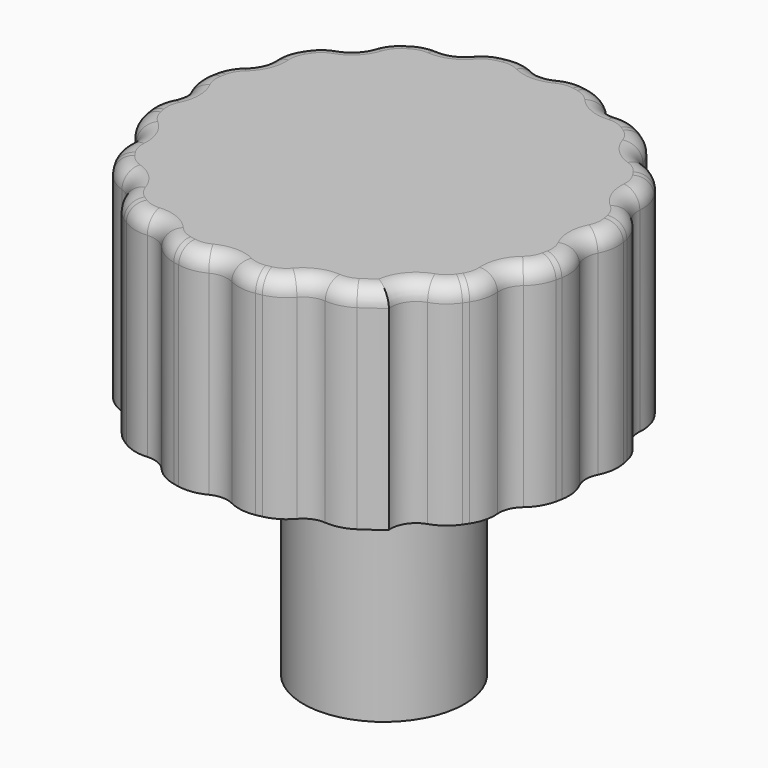
from build123d import *

# Parameters (mm, degrees)
F3_R           = 25
F4_DEPTH       = 25
F5_R           = 9.5
F6_DEPTH       = 28
F8_DEPTH       = 15
F9_R           = 3
F10_DEPTH      = 25
F11_COUNT      = 16
F13_R          = 5
F14_T4_ANGLE   = 1.6121793849
F14_T6_ANGLE   = 53.896069647
F14_T8_ANGLE   = 37.3919452447
F14_T10_ANGLE  = 37.3919452447
F14_T12_ANGLE  = 1.6121793849
F14_T14_ANGLE  = 37.3919452447
F14_T16_ANGLE  = 37.3919452447
F14_T18_ANGLE  = 53.896069647
F14_T20_ANGLE  = 53.896069647
F14_T22_ANGLE  = 37.3919452447
F14_T24_ANGLE  = 37.3919452447
F14_T26_ANGLE  = 1.6121793849
F14_T28_ANGLE  = 1.6121793849
F14_T30_ANGLE  = 37.3919452447
F14_T32_ANGLE  = 37.3919452447
F14_T34_ANGLE  = 53.896069647
F14_T36_ANGLE  = 172.9885237531
F14_T38_ANGLE  = 37.3919452447
F14_T40_ANGLE  = 18.2008968181
F14_T42_ANGLE  = 1.6121793849
F14_T44_ANGLE  = 37.3919452447
F14_T46_ANGLE  = 37.3919452447
F14_T48_ANGLE  = 53.896069647
F14_T50_ANGLE  = 53.896069647
F14_T52_ANGLE  = 37.3919452447
F14_T54_ANGLE  = 37.3919452447
F14_T56_ANGLE  = 1.6121793849
F14_T58_ANGLE  = 1.6121793849
F14_T60_ANGLE  = 37.3919452447
F14_T62_ANGLE  = 37.3919452447
F14_T64_ANGLE  = 53.896069647
F14_T66_ANGLE  = 53.896069647
F14_T68_ANGLE  = 37.3919452447
F14_T70_ANGLE  = 37.3919452447
F14_T72_ANGLE  = 1.6121793849
F14_T74_ANGLE  = 1.6121793849
F14_T76_ANGLE  = 37.3919452447
F14_T78_ANGLE  = 37.3919452447
F14_T80_ANGLE  = 53.896069647
F14_T82_ANGLE  = 53.896069647
F14_T84_ANGLE  = 37.3919452447
F14_T86_ANGLE  = 37.3919452447
F14_T88_ANGLE  = 1.6121793849
F14_T90_ANGLE  = 1.6121793849
F14_T92_ANGLE  = 37.3919452447
F14_T94_ANGLE  = 37.3919452447
F14_T96_ANGLE  = 53.896069647
F14_T98_ANGLE  = 53.896069647
F14_T100_ANGLE = 37.3919452447
F14_T102_ANGLE = 37.3919452447
F14_T104_ANGLE = 1.6121793849
F14_T106_ANGLE = 1.6121793849
F14_T108_ANGLE = 37.3919452447
F14_T110_ANGLE = 37.3919452447
F14_T112_ANGLE = 53.896069647
F14_T114_ANGLE = 53.896069647
F14_T116_ANGLE = 37.3919452447
F14_T118_ANGLE = 37.3919452447
F14_T120_ANGLE = 1.6121793849
F14_T122_ANGLE = 1.6121793849
F14_T124_ANGLE = 37.3919452447
F14_T126_ANGLE = 37.3919452447
F14_T128_ANGLE = 53.896069647


# Not quite as in the source:
# - a fillet or chamfer that OpenCascade refuses, or shapes differently, is made with other operations: its cross-section is extruded or revolved along the edge and cut away or added


with BuildPart() as f4:
    # F3 (on Top) → F4 (new body, through all)
    with BuildSketch(Plane.XY):
        Circle(F3_R)
    extrude(amount=-F4_DEPTH)

    # F5 (on offset) → F6 (join, through all)
    with BuildSketch(Plane.XY.offset(-25)):
        Circle(F5_R)
    extrude(amount=-F6_DEPTH)

    # F7 (on offset) → F8 (cut)
    with BuildSketch(Plane.XY.offset(-53)):
        with BuildLine():
            Line((3.1224989992, 2.5), (-3.1224989992, 2.5))
            ThreePointArc((-3.1224989992, 2.5), (0, -4), (3.1224989992, 2.5))
        make_face()
    extrude(amount=F8_DEPTH, mode=Mode.SUBTRACT)


with BuildPart() as f10:
    # F9 (on Top) → F10 (new body, through all)
    with BuildSketch(Plane.XY):
        with Locations((0, 26.8)):
            Circle(F9_R)
    extrude(amount=-F10_DEPTH)


with BuildPart() as f11_1:
    # F11: instance of F10
    add(f10.part.rotate(Axis((0, 0, 0), (0, 0, 1)), 1 * 360 / F11_COUNT))


with BuildPart() as f11_2:
    # F11: instance of F10
    add(f10.part.rotate(Axis((0, 0, 0), (0, 0, 1)), 2 * 360 / F11_COUNT))


with BuildPart() as f11_3:
    # F11: instance of F10
    add(f10.part.rotate(Axis((0, 0, 0), (0, 0, 1)), 3 * 360 / F11_COUNT))


with BuildPart() as f11_4:
    # F11: instance of F10
    add(f10.part.rotate(Axis((0, 0, 0), (0, 0, 1)), 4 * 360 / F11_COUNT))


with BuildPart() as f11_5:
    # F11: instance of F10
    add(f10.part.rotate(Axis((0, 0, 0), (0, 0, 1)), 5 * 360 / F11_COUNT))


with BuildPart() as f11_6:
    # F11: instance of F10
    add(f10.part.rotate(Axis((0, 0, 0), (0, 0, 1)), 6 * 360 / F11_COUNT))


with BuildPart() as f11_7:
    # F11: instance of F10
    add(f10.part.rotate(Axis((0, 0, 0), (0, 0, 1)), 7 * 360 / F11_COUNT))


with BuildPart() as f11_8:
    # F11: instance of F10
    add(f10.part.rotate(Axis((0, 0, 0), (0, 0, 1)), 8 * 360 / F11_COUNT))


with BuildPart() as f11_9:
    # F11: instance of F10
    add(f10.part.rotate(Axis((0, 0, 0), (0, 0, 1)), 9 * 360 / F11_COUNT))


with BuildPart() as f11_10:
    # F11: instance of F10
    add(f10.part.rotate(Axis((0, 0, 0), (0, 0, 1)), 10 * 360 / F11_COUNT))


with BuildPart() as f11_11:
    # F11: instance of F10
    add(f10.part.rotate(Axis((0, 0, 0), (0, 0, 1)), 11 * 360 / F11_COUNT))


with BuildPart() as f11_12:
    # F11: instance of F10
    add(f10.part.rotate(Axis((0, 0, 0), (0, 0, 1)), 12 * 360 / F11_COUNT))


with BuildPart() as f11_13:
    # F11: instance of F10
    add(f10.part.rotate(Axis((0, 0, 0), (0, 0, 1)), 13 * 360 / F11_COUNT))


with BuildPart() as f11_14:
    # F11: instance of F10
    add(f10.part.rotate(Axis((0, 0, 0), (0, 0, 1)), 14 * 360 / F11_COUNT))


with BuildPart() as f11_15:
    # F11: instance of F10
    add(f10.part.rotate(Axis((0, 0, 0), (0, 0, 1)), 15 * 360 / F11_COUNT))


with BuildPart() as f4_1:
    add(f4.part)

    # F12: cut F10, F11_1, F11_2, F11_3, F11_4, F11_5, F11_6, F11_7, F11_8, F11_9, F11_10, F11_11, F11_12, F11_13, F11_14, F11_15
    add(f10.part, mode=Mode.SUBTRACT)
    add(f11_1.part, mode=Mode.SUBTRACT)
    add(f11_2.part, mode=Mode.SUBTRACT)
    add(f11_3.part, mode=Mode.SUBTRACT)
    add(f11_4.part, mode=Mode.SUBTRACT)
    add(f11_5.part, mode=Mode.SUBTRACT)
    add(f11_6.part, mode=Mode.SUBTRACT)
    add(f11_7.part, mode=Mode.SUBTRACT)
    add(f11_8.part, mode=Mode.SUBTRACT)
    add(f11_9.part, mode=Mode.SUBTRACT)
    add(f11_10.part, mode=Mode.SUBTRACT)
    add(f11_11.part, mode=Mode.SUBTRACT)
    add(f11_12.part, mode=Mode.SUBTRACT)
    add(f11_13.part, mode=Mode.SUBTRACT)
    add(f11_14.part, mode=Mode.SUBTRACT)
    add(f11_15.part, mode=Mode.SUBTRACT)

    # F13
    f13_edges = [f4_1.edges().sort_by_distance(p)[0] for p in [
        (-2.31551, 24.892537, -12.5),
        (2.31551, 24.892537, -12.5),
        (7.386709, 23.883813, -12.5),
        (11.665214, 22.111598, -12.5),
        (15.964369, 19.238995, -12.5),
        (19.238995, 15.964369, -12.5),
        (23.883813, 7.386709, -12.5),
        (22.111598, 11.665214, -12.5),
        (24.892537, 2.31551, -12.5),
        (24.892537, -2.31551, -12.5),
        (23.883813, -7.386709, -12.5),
        (22.111598, -11.665214, -12.5),
        (11.665214, -22.111598, -12.5),
        (7.386709, -23.883813, -12.5),
        (2.31551, -24.892537, -12.5),
        (-2.31551, -24.892537, -12.5),
        (-7.386709, -23.883813, -12.5),
        (-11.665214, -22.111598, -12.5),
        (-15.964369, -19.238995, -12.5),
        (-19.238995, -15.964369, -12.5),
        (-22.111598, -11.665214, -12.5),
        (-23.883813, -7.386709, -12.5),
        (-24.892537, -2.31551, -12.5),
        (-24.892537, 2.31551, -12.5),
        (-23.883813, 7.386709, -12.5),
        (-22.111598, 11.665214, -12.5),
        (-19.238995, 15.964369, -12.5),
        (-15.964369, 19.238995, -12.5),
        (-11.665214, 22.111598, -12.5),
        (-7.386709, 23.883813, -12.5),
        (19.238995, -15.964369, -12.5),
    ]]
    fillet(f13_edges, radius=F13_R)

    # F14: fillet of radius 2 on 64 edges, made by hand

    # F14_s1 → F14_t2 (revolve)
    with BuildSketch(Plane.XZ):
        with BuildLine():
            ThreePointArc((11.5, -25), (10.0857864376, -25.5857864376), (9.5, -27))
            Line((9.5, -27), (9.5, -25))
            Line((9.5, -25), (11.5, -25))
        make_face()
    revolve(axis=Axis((0, 0, -25), (0, 0, 1)))

    # F14_s3 → F14_t4 (revolve, cut)
    with BuildSketch(Plane(origin=(0, 0, 0), x_dir=(0, 0, 1), z_dir=(0.1812728811, -0.9834328358, 0))):
        with BuildLine():
            ThreePointArc((-2, -25), (-0.5857864376, -24.4142135624), (0, -23))
            Line((0, -23), (0, -25))
            Line((0, -25), (-2, -25))
        make_face()
    revolve(axis=Axis((0, 0, 0), (0, 0, 1)), revolution_arc=F14_T4_ANGLE, mode=Mode.SUBTRACT)

    # F14_s5 → F14_t6 (revolve, cut)
    with BuildSketch(Plane(origin=(5.5040261194, 10.8265228248, 0), x_dir=(0, 0, 1), z_dir=(0.4531822028, 0.8914179104, 0))):
        with BuildLine():
            ThreePointArc((0, 18.89), (-0.5857864376, 20.3042135624), (-2, 20.89))
            Line((-2, 20.89), (0, 20.89))
            Line((0, 20.89), (0, 18.89))
        make_face()
    revolve(axis=Axis((26.8, 0, 0), (0, 0, 1)), revolution_arc=F14_T6_ANGLE, mode=Mode.SUBTRACT)

    # F14_s7 → F14_t8 (revolve, cut)
    with BuildSketch(Plane(origin=(4.5e-09, -2.44e-08, 0), x_dir=(0, 0, 1), z_dir=(-0.1812728821, 0.9834328356, 0))):
        with BuildLine():
            ThreePointArc((0, 22.9999999992), (-0.5857864376, 24.4142135616), (-2, 24.9999999992))
            Line((-2, 24.9999999992), (0, 25))
            Line((0, 25), (0, 22.9999999992))
        make_face()
    revolve(axis=Axis((19.6686567317, 3.6254576202, 0), (0, 0, -1)), revolution_arc=F14_T8_ANGLE, mode=Mode.SUBTRACT)

    # F14_s9 → F14_t10 (revolve, cut)
    with BuildSketch(Plane(origin=(5.5040261395, -10.8265228379, 0), x_dir=(0, 0, 1), z_dir=(-0.4531822037, 0.89141791, 0))):
        with BuildLine():
            ThreePointArc((0, 18.8899999871), (-0.5857864376, 20.3042135495), (-2, 20.8899999871))
            Line((-2, 20.8899999871), (0, 20.889999988))
            Line((0, 20.889999988), (0, 18.8899999871))
        make_face()
    revolve(axis=Axis((19.6686567317, -3.6254576202, 0), (0, 0, -1)), revolution_arc=F14_T10_ANGLE, mode=Mode.SUBTRACT)

    # F14_s11 → F14_t12 (revolve, cut)
    with BuildSketch(Plane(origin=(0, 0, 0), x_dir=(0, 0, 1), z_dir=(-0.2088691484, -0.977943597, 0))):
        with BuildLine():
            ThreePointArc((0, -23), (-0.5857864376, -24.4142135624), (-2, -25))
            Line((-2, -25), (0, -25))
            Line((0, -25), (0, -23))
        make_face()
    revolve(axis=Axis((0, 0, 0), (0, 0, 1)), revolution_arc=F14_T12_ANGLE, mode=Mode.SUBTRACT)

    # F14_s13 → F14_t14 (revolve, cut)
    with BuildSketch(Plane(origin=(-5.2e-09, 2.42e-08, 0), x_dir=(0, 0, 1), z_dir=(0.2088691475, -0.9779435972, 0))):
        with BuildLine():
            ThreePointArc((0, -22.9999999992), (-0.5857864376, -24.4142135616), (-2, -24.9999999992))
            Line((-2, -24.9999999992), (0, -25))
            Line((0, -25), (0, -22.9999999992))
        make_face()
    revolve(axis=Axis((19.5588719524, 4.1773829768, 0), (0, 0, 1)), revolution_arc=F14_T14_ANGLE, mode=Mode.SUBTRACT)

    # F14_s15 → F14_t16 (revolve, cut)
    with BuildSketch(Plane(origin=(-5.2e-09, -2.42e-08, 0), x_dir=(0, 0, 1), z_dir=(0.2088691475, 0.9779435972, 0))):
        with BuildLine():
            ThreePointArc((0, 22.9999999992), (-0.5857864376, 24.4142135616), (-2, 24.9999999992))
            Line((-2, 24.9999999992), (0, 25))
            Line((0, 25), (0, 22.9999999992))
        make_face()
    revolve(axis=Axis((19.5588719524, -4.1773829768, 0), (0, 0, -1)), revolution_arc=F14_T16_ANGLE, mode=Mode.SUBTRACT)

    # F14_s17 → F14_t18 (revolve, cut)
    with BuildSketch(Plane(origin=(0.9419261629, 12.1087024533, 0), x_dir=(0, 0, 1), z_dir=(0.077554896, 0.9969880832, 0))):
        with BuildLine():
            ThreePointArc((0, 18.89), (-0.5857864376, 20.3042135624), (-2, 20.89))
            Line((-2, 20.89), (0, 20.89))
            Line((0, 20.89), (0, 18.89))
        make_face()
    revolve(axis=Axis((24.7599714713, 10.2559159874, 0), (0, 0, 1)), revolution_arc=F14_T18_ANGLE, mode=Mode.SUBTRACT)

    # F14_s19 → F14_t20 (revolve, cut)
    with BuildSketch(Plane(origin=(9.2281879933, 7.8961032389, 0), x_dir=(0, 0, 1), z_dir=(0.7598166273, 0.6501374415, 0))):
        with BuildLine():
            ThreePointArc((0, 18.89), (-0.5857864376, 20.3042135624), (-2, 20.89))
            Line((-2, 20.89), (0, 20.89))
            Line((0, 20.89), (0, 18.89))
        make_face()
    revolve(axis=Axis((24.7599714713, -10.2559159874, 0), (0, 0, 1)), revolution_arc=F14_T20_ANGLE, mode=Mode.SUBTRACT)

    # F14_s21 → F14_t22 (revolve, cut)
    with BuildSketch(Plane(origin=(0.9419261765, 12.1087024731, 0), x_dir=(0, 0, 1), z_dir=(-0.077554897, -0.9969880832, 0))):
        with BuildLine():
            ThreePointArc((0, -18.8899999871), (-0.5857864376, -20.3042135495), (-2, -20.8899999871))
            Line((-2, -20.8899999871), (0, -20.889999988))
            Line((0, -20.889999988), (0, -18.8899999871))
        make_face()
    revolve(axis=Axis((16.7840668204, 10.8763551594, 0), (0, 0, 1)), revolution_arc=F14_T22_ANGLE, mode=Mode.SUBTRACT)

    # F14_s23 → F14_t24 (revolve, cut)
    with BuildSketch(Plane(origin=(0.9419261765, -12.1087024731, 0), x_dir=(0, 0, 1), z_dir=(-0.077554897, 0.9969880832, 0))):
        with BuildLine():
            ThreePointArc((0, 18.8899999871), (-0.5857864376, 20.3042135495), (-2, 20.8899999871))
            Line((-2, 20.8899999871), (0, 20.889999988))
            Line((0, 20.889999988), (0, 18.8899999871))
        make_face()
    revolve(axis=Axis((16.7840668204, -10.8763551594, 0), (0, 0, -1)), revolution_arc=F14_T24_ANGLE, mode=Mode.SUBTRACT)

    # F14_s25 → F14_t26 (revolve, cut)
    with BuildSketch(Plane(origin=(0, 0, 0), x_dir=(0, 0, 1), z_dir=(0.5438177578, -0.8392033403, 0))):
        with BuildLine():
            ThreePointArc((0, -23), (-0.5857864376, -24.4142135624), (-2, -25))
            Line((-2, -25), (0, -25))
            Line((0, -25), (0, -23))
        make_face()
    revolve(axis=Axis((0, 0, 0), (0, 0, 1)), revolution_arc=F14_T26_ANGLE, mode=Mode.SUBTRACT)

    # F14_s27 → F14_t28 (revolve, cut)
    with BuildSketch(Plane(origin=(0, 0, 0), x_dir=(0, 0, 1), z_dir=(-0.5672127436, -0.8235713105, 0))):
        with BuildLine():
            ThreePointArc((0, -23), (-0.5857864376, -24.4142135624), (-2, -25))
            Line((-2, -25), (0, -25))
            Line((0, -25), (0, -23))
        make_face()
    revolve(axis=Axis((0, 0, 0), (0, 0, 1)), revolution_arc=F14_T28_ANGLE, mode=Mode.SUBTRACT)

    # F14_s29 → F14_t30 (revolve, cut)
    with BuildSketch(Plane(origin=(11.5474419224, -3.7635735082, 0), x_dir=(0, 0, 1), z_dir=(-0.9507758584, 0.3098794397, 0))):
        with BuildLine():
            ThreePointArc((0, 18.8899999871), (-0.5857864376, 20.3042135495), (-2, 20.8899999871))
            Line((-2, 20.8899999871), (0, 20.889999988))
            Line((0, 20.889999988), (0, 18.8899999871))
        make_face()
    revolve(axis=Axis((16.47142622, 11.3442548837, 0), (0, 0, -1)), revolution_arc=F14_T30_ANGLE, mode=Mode.SUBTRACT)

    # F14_s31 → F14_t32 (revolve, cut)
    with BuildSketch(Plane(origin=(-1.41e-08, -2.04e-08, 0), x_dir=(0, 0, 1), z_dir=(0.5672127427, 0.8235713111, 0))):
        with BuildLine():
            ThreePointArc((0, 22.9999999992), (-0.5857864376, 24.4142135616), (-2, 24.9999999992))
            Line((-2, 24.9999999992), (0, 25))
            Line((0, 25), (0, 22.9999999992))
        make_face()
    revolve(axis=Axis((16.47142622, -11.3442548837, 0), (0, 0, -1)), revolution_arc=F14_T32_ANGLE, mode=Mode.SUBTRACT)

    # F14_s33 → F14_t34 (revolve, cut)
    with BuildSketch(Plane(origin=(-3.7635735133, 11.547441899, 0), x_dir=(0, 0, 1), z_dir=(-0.3098794406, 0.9507758581, 0))):
        with BuildLine():
            ThreePointArc((0, 18.89), (-0.5857864376, 20.3042135624), (-2, 20.89))
            Line((-2, 20.89), (0, 20.89))
            Line((0, 20.89), (0, 18.89))
        make_face()
    revolve(axis=Axis((18.9504617358, 18.9504617358, 0), (0, 0, 1)), revolution_arc=F14_T34_ANGLE, mode=Mode.SUBTRACT)

    # F14_s35 → F14_t36 (revolve, cut)
    with BuildSketch(Plane(origin=(11.547441899, 3.7635735133, 0), x_dir=(0, 0, 1), z_dir=(0.9507758581, 0.3098794406, 0))):
        with BuildLine():
            ThreePointArc((0, 18.89), (-0.5857864376, 20.3042135624), (-2, 20.89))
            Line((-2, 20.89), (0, 20.89))
            Line((0, 20.89), (0, 18.89))
        make_face()
    revolve(axis=Axis((18.9504617358, -18.9504617358, 0), (0, 0, 1)), revolution_arc=F14_T36_ANGLE, mode=Mode.SUBTRACT)

    # F14_s37 → F14_t38 (revolve, cut)
    with BuildSketch(Plane(origin=(2.04e-08, -1.41e-08, 0), x_dir=(0, 0, 1), z_dir=(-0.8235713111, 0.5672127427, 0))):
        with BuildLine():
            ThreePointArc((0, 22.9999999992), (-0.5857864376, 24.4142135616), (-2, 24.9999999992))
            Line((-2, 24.9999999992), (0, 25))
            Line((0, 25), (0, 22.9999999992))
        make_face()
    revolve(axis=Axis((11.3442548837, 16.47142622, 0), (0, 0, -1)), revolution_arc=F14_T38_ANGLE, mode=Mode.SUBTRACT)

    # F14_s39 → F14_t40 (revolve, cut)
    with BuildSketch(Plane(origin=(0, 0, 0), x_dir=(0, 0, 1), z_dir=(-0.8392033403, -0.5438177578, 0))):
        with BuildLine():
            ThreePointArc((0, -23), (-0.5857864376, -24.4142135624), (-2, -25))
            Line((-2, -25), (0, -25))
            Line((0, -25), (0, -23))
        make_face()
    revolve(axis=Axis((0, 0, 0), (0, 0, 1)), revolution_arc=F14_T40_ANGLE, mode=Mode.SUBTRACT)

    # F14_s41 → F14_t42 (revolve, cut)
    with BuildSketch(Plane(origin=(0, 0, 0), x_dir=(0, 0, 1), z_dir=(0.8235713105, -0.5672127436, 0))):
        with BuildLine():
            ThreePointArc((0, -23), (-0.5857864376, -24.4142135624), (-2, -25))
            Line((-2, -25), (0, -25))
            Line((0, -25), (0, -23))
        make_face()
    revolve(axis=Axis((0, 0, 0), (0, 0, 1)), revolution_arc=F14_T42_ANGLE, mode=Mode.SUBTRACT)

    # F14_s43 → F14_t44 (revolve, cut)
    with BuildSketch(Plane(origin=(-2.08e-08, -1.35e-08, 0), x_dir=(0, 0, 1), z_dir=(0.8392033397, 0.5438177586, 0))):
        with BuildLine():
            ThreePointArc((0, 22.9999999992), (-0.5857864376, 24.4142135616), (-2, 24.9999999992))
            Line((-2, 24.9999999992), (0, 25))
            Line((0, 25), (0, 22.9999999992))
        make_face()
    revolve(axis=Axis((10.8763551594, -16.7840668204, 0), (0, 0, -1)), revolution_arc=F14_T44_ANGLE, mode=Mode.SUBTRACT)

    # F14_s45 → F14_t46 (revolve, cut)
    with BuildSketch(Plane(origin=(12.1087024731, 0.9419261765, 0), x_dir=(0, 0, 1), z_dir=(-0.9969880832, -0.077554897, 0))):
        with BuildLine():
            ThreePointArc((0, 18.8899999871), (-0.5857864376, 20.3042135495), (-2, 20.8899999871))
            Line((-2, 20.8899999871), (0, 20.889999988))
            Line((0, 20.889999988), (0, 18.8899999871))
        make_face()
    revolve(axis=Axis((10.8763551594, 16.7840668204, 0), (0, 0, -1)), revolution_arc=F14_T46_ANGLE, mode=Mode.SUBTRACT)

    # F14_s47 → F14_t48 (revolve, cut)
    with BuildSketch(Plane(origin=(12.1087024533, -0.9419261629, 0), x_dir=(0, 0, 1), z_dir=(0.9969880832, -0.077554896, 0))):
        with BuildLine():
            ThreePointArc((0, 18.89), (-0.5857864376, 20.3042135624), (-2, 20.89))
            Line((-2, 20.89), (0, 20.89))
            Line((0, 20.89), (0, 18.89))
        make_face()
    revolve(axis=Axis((10.2559159874, -24.7599714713, 0), (0, 0, 1)), revolution_arc=F14_T48_ANGLE, mode=Mode.SUBTRACT)

    # F14_s49 → F14_t50 (revolve, cut)
    with BuildSketch(Plane(origin=(-7.8961032389, 9.2281879933, 0), x_dir=(0, 0, 1), z_dir=(-0.6501374415, 0.7598166273, 0))):
        with BuildLine():
            ThreePointArc((0, 18.89), (-0.5857864376, 20.3042135624), (-2, 20.89))
            Line((-2, 20.89), (0, 20.89))
            Line((0, 20.89), (0, 18.89))
        make_face()
    revolve(axis=Axis((10.2559159874, 24.7599714713, 0), (0, 0, 1)), revolution_arc=F14_T50_ANGLE, mode=Mode.SUBTRACT)

    # F14_s51 → F14_t52 (revolve, cut)
    with BuildSketch(Plane(origin=(-7.8961032433, -9.2281880169, 0), x_dir=(0, 0, 1), z_dir=(0.6501374408, 0.7598166279, 0))):
        with BuildLine():
            ThreePointArc((0, 18.8899999871), (-0.5857864376, 20.3042135495), (-2, 20.8899999871))
            Line((-2, 20.8899999871), (0, 20.889999988))
            Line((0, 20.889999988), (0, 18.8899999871))
        make_face()
    revolve(axis=Axis((4.1773829768, -19.5588719524, 0), (0, 0, -1)), revolution_arc=F14_T52_ANGLE, mode=Mode.SUBTRACT)

    # F14_s53 → F14_t54 (revolve, cut)
    with BuildSketch(Plane(origin=(2.42e-08, -5.2e-09, 0), x_dir=(0, 0, 1), z_dir=(-0.9779435972, 0.2088691475, 0))):
        with BuildLine():
            ThreePointArc((0, 22.9999999992), (-0.5857864376, 24.4142135616), (-2, 24.9999999992))
            Line((-2, 24.9999999992), (0, 25))
            Line((0, 25), (0, 22.9999999992))
        make_face()
    revolve(axis=Axis((4.1773829768, 19.5588719524, 0), (0, 0, -1)), revolution_arc=F14_T54_ANGLE, mode=Mode.SUBTRACT)

    # F14_s55 → F14_t56 (revolve, cut)
    with BuildSketch(Plane(origin=(0, 0, 0), x_dir=(0, 0, 1), z_dir=(-0.9834328358, -0.1812728811, 0))):
        with BuildLine():
            ThreePointArc((0, -23), (-0.5857864376, -24.4142135624), (-2, -25))
            Line((-2, -25), (0, -25))
            Line((0, -25), (0, -23))
        make_face()
    revolve(axis=Axis((0, 0, 0), (0, 0, 1)), revolution_arc=F14_T56_ANGLE, mode=Mode.SUBTRACT)

    # F14_s57 → F14_t58 (revolve, cut)
    with BuildSketch(Plane(origin=(0, 0, 0), x_dir=(0, 0, 1), z_dir=(0.977943597, -0.2088691484, 0))):
        with BuildLine():
            ThreePointArc((0, -23), (-0.5857864376, -24.4142135624), (-2, -25))
            Line((-2, -25), (0, -25))
            Line((0, -25), (0, -23))
        make_face()
    revolve(axis=Axis((0, 0, 0), (0, 0, 1)), revolution_arc=F14_T58_ANGLE, mode=Mode.SUBTRACT)

    # F14_s59 → F14_t60 (revolve, cut)
    with BuildSketch(Plane(origin=(-2.44e-08, -4.5e-09, 0), x_dir=(0, 0, 1), z_dir=(0.9834328356, 0.1812728821, 0))):
        with BuildLine():
            ThreePointArc((0, 22.9999999992), (-0.5857864376, 24.4142135616), (-2, 24.9999999992))
            Line((-2, 24.9999999992), (0, 25))
            Line((0, 25), (0, 22.9999999992))
        make_face()
    revolve(axis=Axis((3.6254576202, -19.6686567317, 0), (0, 0, -1)), revolution_arc=F14_T60_ANGLE, mode=Mode.SUBTRACT)

    # F14_s61 → F14_t62 (revolve, cut)
    with BuildSketch(Plane(origin=(10.8265228379, 5.5040261395, 0), x_dir=(0, 0, 1), z_dir=(-0.89141791, -0.4531822037, 0))):
        with BuildLine():
            ThreePointArc((0, 18.8899999871), (-0.5857864376, 20.3042135495), (-2, 20.8899999871))
            Line((-2, 20.8899999871), (0, 20.889999988))
            Line((0, 20.889999988), (0, 18.8899999871))
        make_face()
    revolve(axis=Axis((3.6254576202, 19.6686567317, 0), (0, 0, -1)), revolution_arc=F14_T62_ANGLE, mode=Mode.SUBTRACT)

    # F14_s63 → F14_t64 (revolve, cut)
    with BuildSketch(Plane(origin=(10.8265228248, -5.5040261194, 0), x_dir=(0, 0, 1), z_dir=(0.8914179104, -0.4531822028, 0))):
        with BuildLine():
            ThreePointArc((0, 18.89), (-0.5857864376, 20.3042135624), (-2, 20.89))
            Line((-2, 20.89), (0, 20.89))
            Line((0, 20.89), (0, 18.89))
        make_face()
    revolve(axis=Axis((0, -26.8, 0), (0, 0, 1)), revolution_arc=F14_T64_ANGLE, mode=Mode.SUBTRACT)

    # F14_s65 → F14_t66 (revolve, cut)
    with BuildSketch(Plane(origin=(-10.8265228248, 5.5040261194, 0), x_dir=(0, 0, 1), z_dir=(-0.8914179104, 0.4531822028, 0))):
        with BuildLine():
            ThreePointArc((0, 18.89), (-0.5857864376, 20.3042135624), (-2, 20.89))
            Line((-2, 20.89), (0, 20.89))
            Line((0, 20.89), (0, 18.89))
        make_face()
    revolve(axis=Axis((0, 26.8, 0), (0, 0, 1)), revolution_arc=F14_T66_ANGLE, mode=Mode.SUBTRACT)

    # F14_s67 → F14_t68 (revolve, cut)
    with BuildSketch(Plane(origin=(-10.8265228379, -5.5040261395, 0), x_dir=(0, 0, 1), z_dir=(0.89141791, 0.4531822037, 0))):
        with BuildLine():
            ThreePointArc((0, 18.8899999871), (-0.5857864376, 20.3042135495), (-2, 20.8899999871))
            Line((-2, 20.8899999871), (0, 20.889999988))
            Line((0, 20.889999988), (0, 18.8899999871))
        make_face()
    revolve(axis=Axis((-3.6254576202, -19.6686567317, 0), (0, 0, -1)), revolution_arc=F14_T68_ANGLE, mode=Mode.SUBTRACT)

    # F14_s69 → F14_t70 (revolve, cut)
    with BuildSketch(Plane(origin=(2.44e-08, 4.5e-09, 0), x_dir=(0, 0, 1), z_dir=(-0.9834328356, -0.1812728821, 0))):
        with BuildLine():
            ThreePointArc((0, 22.9999999992), (-0.5857864376, 24.4142135616), (-2, 24.9999999992))
            Line((-2, 24.9999999992), (0, 25))
            Line((0, 25), (0, 22.9999999992))
        make_face()
    revolve(axis=Axis((-3.6254576202, 19.6686567317, 0), (0, 0, -1)), revolution_arc=F14_T70_ANGLE, mode=Mode.SUBTRACT)

    # F14_s71 → F14_t72 (revolve, cut)
    with BuildSketch(Plane(origin=(0, 0, 0), x_dir=(0, 0, 1), z_dir=(-0.977943597, 0.2088691484, 0))):
        with BuildLine():
            ThreePointArc((0, -23), (-0.5857864376, -24.4142135624), (-2, -25))
            Line((-2, -25), (0, -25))
            Line((0, -25), (0, -23))
        make_face()
    revolve(axis=Axis((0, 0, 0), (0, 0, 1)), revolution_arc=F14_T72_ANGLE, mode=Mode.SUBTRACT)

    # F14_s73 → F14_t74 (revolve, cut)
    with BuildSketch(Plane(origin=(0, 0, 0), x_dir=(0, 0, 1), z_dir=(0.9834328358, 0.1812728811, 0))):
        with BuildLine():
            ThreePointArc((0, -23), (-0.5857864376, -24.4142135624), (-2, -25))
            Line((-2, -25), (0, -25))
            Line((0, -25), (0, -23))
        make_face()
    revolve(axis=Axis((0, 0, 0), (0, 0, 1)), revolution_arc=F14_T74_ANGLE, mode=Mode.SUBTRACT)

    # F14_s75 → F14_t76 (revolve, cut)
    with BuildSketch(Plane(origin=(-2.42e-08, 5.2e-09, 0), x_dir=(0, 0, 1), z_dir=(0.9779435972, -0.2088691475, 0))):
        with BuildLine():
            ThreePointArc((0, 22.9999999992), (-0.5857864376, 24.4142135616), (-2, 24.9999999992))
            Line((-2, 24.9999999992), (0, 25))
            Line((0, 25), (0, 22.9999999992))
        make_face()
    revolve(axis=Axis((-4.1773829768, -19.5588719524, 0), (0, 0, -1)), revolution_arc=F14_T76_ANGLE, mode=Mode.SUBTRACT)

    # F14_s77 → F14_t78 (revolve, cut)
    with BuildSketch(Plane(origin=(7.8961032433, 9.2281880169, 0), x_dir=(0, 0, 1), z_dir=(-0.6501374408, -0.7598166279, 0))):
        with BuildLine():
            ThreePointArc((0, 18.8899999871), (-0.5857864376, 20.3042135495), (-2, 20.8899999871))
            Line((-2, 20.8899999871), (0, 20.889999988))
            Line((0, 20.889999988), (0, 18.8899999871))
        make_face()
    revolve(axis=Axis((-4.1773829768, 19.5588719524, 0), (0, 0, -1)), revolution_arc=F14_T78_ANGLE, mode=Mode.SUBTRACT)

    # F14_s79 → F14_t80 (revolve, cut)
    with BuildSketch(Plane(origin=(7.8961032389, -9.2281879933, 0), x_dir=(0, 0, 1), z_dir=(0.6501374415, -0.7598166273, 0))):
        with BuildLine():
            ThreePointArc((0, 18.89), (-0.5857864376, 20.3042135624), (-2, 20.89))
            Line((-2, 20.89), (0, 20.89))
            Line((0, 20.89), (0, 18.89))
        make_face()
    revolve(axis=Axis((-10.2559159874, -24.7599714713, 0), (0, 0, 1)), revolution_arc=F14_T80_ANGLE, mode=Mode.SUBTRACT)

    # F14_s81 → F14_t82 (revolve, cut)
    with BuildSketch(Plane(origin=(-12.1087024533, 0.9419261629, 0), x_dir=(0, 0, 1), z_dir=(-0.9969880832, 0.077554896, 0))):
        with BuildLine():
            ThreePointArc((0, 18.89), (-0.5857864376, 20.3042135624), (-2, 20.89))
            Line((-2, 20.89), (0, 20.89))
            Line((0, 20.89), (0, 18.89))
        make_face()
    revolve(axis=Axis((-10.2559159874, 24.7599714713, 0), (0, 0, 1)), revolution_arc=F14_T82_ANGLE, mode=Mode.SUBTRACT)

    # F14_s83 → F14_t84 (revolve, cut)
    with BuildSketch(Plane(origin=(-12.1087024731, -0.9419261765, 0), x_dir=(0, 0, 1), z_dir=(0.9969880832, 0.077554897, 0))):
        with BuildLine():
            ThreePointArc((0, 18.8899999871), (-0.5857864376, 20.3042135495), (-2, 20.8899999871))
            Line((-2, 20.8899999871), (0, 20.889999988))
            Line((0, 20.889999988), (0, 18.8899999871))
        make_face()
    revolve(axis=Axis((-10.8763551594, -16.7840668204, 0), (0, 0, -1)), revolution_arc=F14_T84_ANGLE, mode=Mode.SUBTRACT)

    # F14_s85 → F14_t86 (revolve, cut)
    with BuildSketch(Plane(origin=(2.08e-08, 1.35e-08, 0), x_dir=(0, 0, 1), z_dir=(-0.8392033397, -0.5438177586, 0))):
        with BuildLine():
            ThreePointArc((0, 22.9999999992), (-0.5857864376, 24.4142135616), (-2, 24.9999999992))
            Line((-2, 24.9999999992), (0, 25))
            Line((0, 25), (0, 22.9999999992))
        make_face()
    revolve(axis=Axis((-10.8763551594, 16.7840668204, 0), (0, 0, -1)), revolution_arc=F14_T86_ANGLE, mode=Mode.SUBTRACT)

    # F14_s87 → F14_t88 (revolve, cut)
    with BuildSketch(Plane(origin=(0, 0, 0), x_dir=(0, 0, 1), z_dir=(-0.8235713105, 0.5672127436, 0))):
        with BuildLine():
            ThreePointArc((0, -23), (-0.5857864376, -24.4142135624), (-2, -25))
            Line((-2, -25), (0, -25))
            Line((0, -25), (0, -23))
        make_face()
    revolve(axis=Axis((0, 0, 0), (0, 0, 1)), revolution_arc=F14_T88_ANGLE, mode=Mode.SUBTRACT)

    # F14_s89 → F14_t90 (revolve, cut)
    with BuildSketch(Plane(origin=(0, 0, 0), x_dir=(0, 0, 1), z_dir=(0.8392033403, 0.5438177578, 0))):
        with BuildLine():
            ThreePointArc((0, -23), (-0.5857864376, -24.4142135624), (-2, -25))
            Line((-2, -25), (0, -25))
            Line((0, -25), (0, -23))
        make_face()
    revolve(axis=Axis((0, 0, 0), (0, 0, 1)), revolution_arc=F14_T90_ANGLE, mode=Mode.SUBTRACT)

    # F14_s91 → F14_t92 (revolve, cut)
    with BuildSketch(Plane(origin=(-2.04e-08, 1.41e-08, 0), x_dir=(0, 0, 1), z_dir=(0.8235713111, -0.5672127427, 0))):
        with BuildLine():
            ThreePointArc((0, 22.9999999992), (-0.5857864376, 24.4142135616), (-2, 24.9999999992))
            Line((-2, 24.9999999992), (0, 25))
            Line((0, 25), (0, 22.9999999992))
        make_face()
    revolve(axis=Axis((-11.3442548837, -16.47142622, 0), (0, 0, -1)), revolution_arc=F14_T92_ANGLE, mode=Mode.SUBTRACT)

    # F14_s93 → F14_t94 (revolve, cut)
    with BuildSketch(Plane(origin=(3.7635735082, 11.5474419224, 0), x_dir=(0, 0, 1), z_dir=(-0.3098794397, -0.9507758584, 0))):
        with BuildLine():
            ThreePointArc((0, 18.8899999871), (-0.5857864376, 20.3042135495), (-2, 20.8899999871))
            Line((-2, 20.8899999871), (0, 20.889999988))
            Line((0, 20.889999988), (0, 18.8899999871))
        make_face()
    revolve(axis=Axis((-11.3442548837, 16.47142622, 0), (0, 0, -1)), revolution_arc=F14_T94_ANGLE, mode=Mode.SUBTRACT)

    # F14_s95 → F14_t96 (revolve, cut)
    with BuildSketch(Plane(origin=(3.7635735133, -11.547441899, 0), x_dir=(0, 0, 1), z_dir=(0.3098794406, -0.9507758581, 0))):
        with BuildLine():
            ThreePointArc((0, 18.89), (-0.5857864376, 20.3042135624), (-2, 20.89))
            Line((-2, 20.89), (0, 20.89))
            Line((0, 20.89), (0, 18.89))
        make_face()
    revolve(axis=Axis((-18.9504617358, -18.9504617358, 0), (0, 0, 1)), revolution_arc=F14_T96_ANGLE, mode=Mode.SUBTRACT)

    # F14_s97 → F14_t98 (revolve, cut)
    with BuildSketch(Plane(origin=(-11.547441899, -3.7635735133, 0), x_dir=(0, 0, 1), z_dir=(-0.9507758581, -0.3098794406, 0))):
        with BuildLine():
            ThreePointArc((0, 18.89), (-0.5857864376, 20.3042135624), (-2, 20.89))
            Line((-2, 20.89), (0, 20.89))
            Line((0, 20.89), (0, 18.89))
        make_face()
    revolve(axis=Axis((-18.9504617358, 18.9504617358, 0), (0, 0, 1)), revolution_arc=F14_T98_ANGLE, mode=Mode.SUBTRACT)

    # F14_s99 → F14_t100 (revolve, cut)
    with BuildSketch(Plane(origin=(-11.5474419224, 3.7635735082, 0), x_dir=(0, 0, 1), z_dir=(0.9507758584, -0.3098794397, 0))):
        with BuildLine():
            ThreePointArc((0, 18.8899999871), (-0.5857864376, 20.3042135495), (-2, 20.8899999871))
            Line((-2, 20.8899999871), (0, 20.889999988))
            Line((0, 20.889999988), (0, 18.8899999871))
        make_face()
    revolve(axis=Axis((-16.47142622, -11.3442548837, 0), (0, 0, -1)), revolution_arc=F14_T100_ANGLE, mode=Mode.SUBTRACT)

    # F14_s101 → F14_t102 (revolve, cut)
    with BuildSketch(Plane(origin=(1.41e-08, 2.04e-08, 0), x_dir=(0, 0, 1), z_dir=(-0.5672127427, -0.8235713111, 0))):
        with BuildLine():
            ThreePointArc((0, 22.9999999992), (-0.5857864376, 24.4142135616), (-2, 24.9999999992))
            Line((-2, 24.9999999992), (0, 25))
            Line((0, 25), (0, 22.9999999992))
        make_face()
    revolve(axis=Axis((-16.47142622, 11.3442548837, 0), (0, 0, -1)), revolution_arc=F14_T102_ANGLE, mode=Mode.SUBTRACT)

    # F14_s103 → F14_t104 (revolve, cut)
    with BuildSketch(Plane(origin=(0, 0, 0), x_dir=(0, 0, 1), z_dir=(-0.5438177578, 0.8392033403, 0))):
        with BuildLine():
            ThreePointArc((0, -23), (-0.5857864376, -24.4142135624), (-2, -25))
            Line((-2, -25), (0, -25))
            Line((0, -25), (0, -23))
        make_face()
    revolve(axis=Axis((0, 0, 0), (0, 0, 1)), revolution_arc=F14_T104_ANGLE, mode=Mode.SUBTRACT)

    # F14_s105 → F14_t106 (revolve, cut)
    with BuildSketch(Plane(origin=(0, 0, 0), x_dir=(0, 0, 1), z_dir=(0.5672127436, 0.8235713105, 0))):
        with BuildLine():
            ThreePointArc((0, -23), (-0.5857864376, -24.4142135624), (-2, -25))
            Line((-2, -25), (0, -25))
            Line((0, -25), (0, -23))
        make_face()
    revolve(axis=Axis((0, 0, 0), (0, 0, 1)), revolution_arc=F14_T106_ANGLE, mode=Mode.SUBTRACT)

    # F14_s107 → F14_t108 (revolve, cut)
    with BuildSketch(Plane(origin=(-1.35e-08, 2.08e-08, 0), x_dir=(0, 0, 1), z_dir=(0.5438177586, -0.8392033397, 0))):
        with BuildLine():
            ThreePointArc((0, 22.9999999992), (-0.5857864376, 24.4142135616), (-2, 24.9999999992))
            Line((-2, 24.9999999992), (0, 25))
            Line((0, 25), (0, 22.9999999992))
        make_face()
    revolve(axis=Axis((-16.7840668204, -10.8763551594, 0), (0, 0, -1)), revolution_arc=F14_T108_ANGLE, mode=Mode.SUBTRACT)

    # F14_s109 → F14_t110 (revolve, cut)
    with BuildSketch(Plane(origin=(-0.9419261765, 12.1087024731, 0), x_dir=(0, 0, 1), z_dir=(0.077554897, -0.9969880832, 0))):
        with BuildLine():
            ThreePointArc((0, 18.8899999871), (-0.5857864376, 20.3042135495), (-2, 20.8899999871))
            Line((-2, 20.8899999871), (0, 20.889999988))
            Line((0, 20.889999988), (0, 18.8899999871))
        make_face()
    revolve(axis=Axis((-16.7840668204, 10.8763551594, 0), (0, 0, -1)), revolution_arc=F14_T110_ANGLE, mode=Mode.SUBTRACT)

    # F14_s111 → F14_t112 (revolve, cut)
    with BuildSketch(Plane(origin=(-0.9419261629, -12.1087024533, 0), x_dir=(0, 0, 1), z_dir=(-0.077554896, -0.9969880832, 0))):
        with BuildLine():
            ThreePointArc((0, 18.89), (-0.5857864376, 20.3042135624), (-2, 20.89))
            Line((-2, 20.89), (0, 20.89))
            Line((0, 20.89), (0, 18.89))
        make_face()
    revolve(axis=Axis((-24.7599714713, -10.2559159874, 0), (0, 0, 1)), revolution_arc=F14_T112_ANGLE, mode=Mode.SUBTRACT)

    # F14_s113 → F14_t114 (revolve, cut)
    with BuildSketch(Plane(origin=(-9.2281879933, -7.8961032389, 0), x_dir=(0, 0, 1), z_dir=(-0.7598166273, -0.6501374415, 0))):
        with BuildLine():
            ThreePointArc((0, 18.89), (-0.5857864376, 20.3042135624), (-2, 20.89))
            Line((-2, 20.89), (0, 20.89))
            Line((0, 20.89), (0, 18.89))
        make_face()
    revolve(axis=Axis((-24.7599714713, 10.2559159874, 0), (0, 0, 1)), revolution_arc=F14_T114_ANGLE, mode=Mode.SUBTRACT)

    # F14_s115 → F14_t116 (revolve, cut)
    with BuildSketch(Plane(origin=(-9.2281880169, 7.8961032433, 0), x_dir=(0, 0, 1), z_dir=(0.7598166279, -0.6501374408, 0))):
        with BuildLine():
            ThreePointArc((0, 18.8899999871), (-0.5857864376, 20.3042135495), (-2, 20.8899999871))
            Line((-2, 20.8899999871), (0, 20.889999988))
            Line((0, 20.889999988), (0, 18.8899999871))
        make_face()
    revolve(axis=Axis((-19.5588719524, -4.1773829768, 0), (0, 0, -1)), revolution_arc=F14_T116_ANGLE, mode=Mode.SUBTRACT)

    # F14_s117 → F14_t118 (revolve, cut)
    with BuildSketch(Plane(origin=(5.2e-09, 2.42e-08, 0), x_dir=(0, 0, 1), z_dir=(-0.2088691475, -0.9779435972, 0))):
        with BuildLine():
            ThreePointArc((0, 22.9999999992), (-0.5857864376, 24.4142135616), (-2, 24.9999999992))
            Line((-2, 24.9999999992), (0, 25))
            Line((0, 25), (0, 22.9999999992))
        make_face()
    revolve(axis=Axis((-19.5588719524, 4.1773829768, 0), (0, 0, -1)), revolution_arc=F14_T118_ANGLE, mode=Mode.SUBTRACT)

    # F14_s119 → F14_t120 (revolve, cut)
    with BuildSketch(Plane(origin=(0, 0, 0), x_dir=(0, 0, 1), z_dir=(-0.1812728811, 0.9834328358, 0))):
        with BuildLine():
            ThreePointArc((0, -23), (-0.5857864376, -24.4142135624), (-2, -25))
            Line((-2, -25), (0, -25))
            Line((0, -25), (0, -23))
        make_face()
    revolve(axis=Axis((0, 0, 0), (0, 0, 1)), revolution_arc=F14_T120_ANGLE, mode=Mode.SUBTRACT)

    # F14_s121 → F14_t122 (revolve, cut)
    with BuildSketch(Plane(origin=(0, 0, 0), x_dir=(0, 0, 1), z_dir=(0.2088691484, 0.977943597, 0))):
        with BuildLine():
            ThreePointArc((0, -23), (-0.5857864376, -24.4142135624), (-2, -25))
            Line((-2, -25), (0, -25))
            Line((0, -25), (0, -23))
        make_face()
    revolve(axis=Axis((0, 0, 0), (0, 0, 1)), revolution_arc=F14_T122_ANGLE, mode=Mode.SUBTRACT)

    # F14_s123 → F14_t124 (revolve, cut)
    with BuildSketch(Plane(origin=(-4.5e-09, 2.44e-08, 0), x_dir=(0, 0, 1), z_dir=(0.1812728821, -0.9834328356, 0))):
        with BuildLine():
            ThreePointArc((0, 22.9999999992), (-0.5857864376, 24.4142135616), (-2, 24.9999999992))
            Line((-2, 24.9999999992), (0, 25))
            Line((0, 25), (0, 22.9999999992))
        make_face()
    revolve(axis=Axis((-19.6686567317, -3.6254576202, 0), (0, 0, -1)), revolution_arc=F14_T124_ANGLE, mode=Mode.SUBTRACT)

    # F14_s125 → F14_t126 (revolve, cut)
    with BuildSketch(Plane(origin=(-5.5040261395, 10.8265228379, 0), x_dir=(0, 0, 1), z_dir=(0.4531822037, -0.89141791, 0))):
        with BuildLine():
            ThreePointArc((0, 18.8899999871), (-0.5857864376, 20.3042135495), (-2, 20.8899999871))
            Line((-2, 20.8899999871), (0, 20.889999988))
            Line((0, 20.889999988), (0, 18.8899999871))
        make_face()
    revolve(axis=Axis((-19.6686567317, 3.6254576202, 0), (0, 0, -1)), revolution_arc=F14_T126_ANGLE, mode=Mode.SUBTRACT)

    # F14_s127 → F14_t128 (revolve, cut)
    with BuildSketch(Plane(origin=(-5.5040261194, -10.8265228248, 0), x_dir=(0, 0, 1), z_dir=(-0.4531822028, -0.8914179104, 0))):
        with BuildLine():
            ThreePointArc((0, 18.89), (-0.5857864376, 20.3042135624), (-2, 20.89))
            Line((-2, 20.89), (0, 20.89))
            Line((0, 20.89), (0, 18.89))
        make_face()
    revolve(axis=Axis((-26.8, 0, 0), (0, 0, 1)), revolution_arc=F14_T128_ANGLE, mode=Mode.SUBTRACT)


solid = f4_1.part
